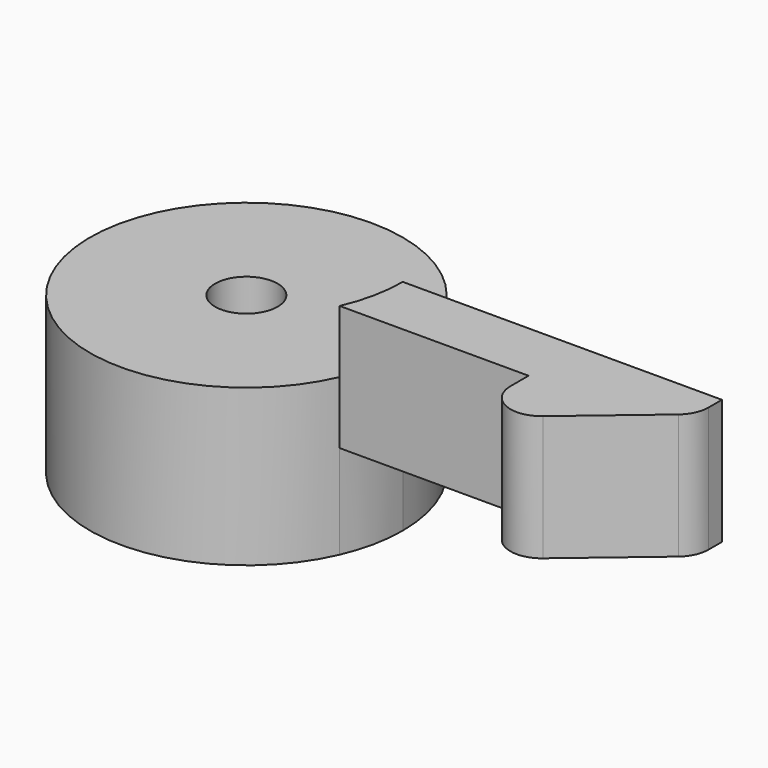
from build123d import *

# Parameters (mm, degrees)
F1_DEPTH = 5
F2_DEPTH = 2
F3_DEPTH = 2
F4_R     = 1
F5_D     = 2


with BuildPart() as f1:
    # F0 (on Top) → F1 (new body)
    with BuildSketch(Plane.XY):
        with BuildLine():
            ThreePointArc((4.582575695, -2), (4.8945315647, -1.0215482184), (5, 0))
            ThreePointArc((5, 0), (-4.8945315647, 1.0215482184), (4.582575695, -2))
        make_face()
    extrude(amount=-F1_DEPTH)

    # F0 (on Top) → F2 (join)
    with BuildSketch(Plane.XY):
        with BuildLine():
            Line((13, 0), (5, 0))
            ThreePointArc((5, 0), (4.8945315647, -1.0215482184), (4.582575695, -2))
            Line((4.582575695, -2), (10.6197060227, -2))
            Line((10.6197060227, -2), (10.6197060227, -4.87568))
            Line((10.6197060227, -4.87568), (15.2, -0.999998501))
            Line((15.2, -0.999998501), (15.2, 0))
            Line((15.2, 0), (13, 0))
        make_face()
    extrude(amount=-F2_DEPTH)

    # F0 (on Top) → F3 (join, symmetric)
    with BuildSketch(Plane.XY):
        with BuildLine():
            Line((13, 0), (5, 0))
            ThreePointArc((5, 0), (4.8945315647, -1.0215482184), (4.582575695, -2))
            Line((4.582575695, -2), (10.6197060227, -2))
            Line((10.6197060227, -2), (10.6197060227, -4.87568))
            Line((10.6197060227, -4.87568), (15.2, -0.999998501))
            Line((15.2, -0.999998501), (15.2, 0))
            Line((15.2, 0), (13, 0))
        make_face()
    extrude(amount=F3_DEPTH, both=True)

    # F4
    f4_edges = [f1.edges().sort_by_distance(p)[0] for p in [
        (10.619706, -4.87568, 0),
        (15.2, -0.999999, 0),
    ]]
    fillet(f4_edges, radius=F4_R)

    # F5 (through all)
    with Locations(Plane.XY):
        with Locations((0, 0)):
            Hole(F5_D / 2)


solid = f1.part
